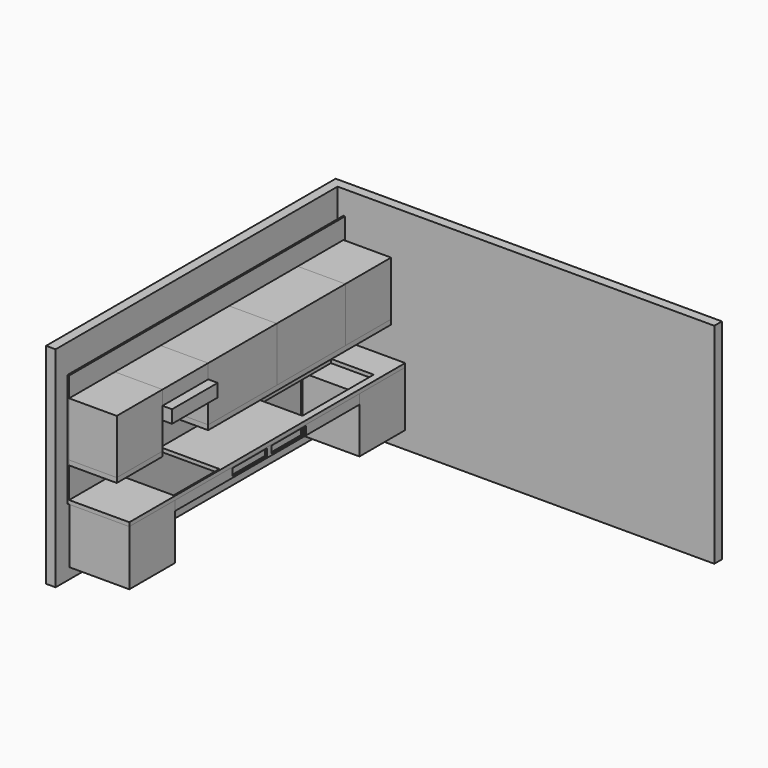
from build123d import *

# Parameters (mm, degrees)
F0_W      = 100
F0_H      = 3700
F1_DEPTH  = 2200
F2_W      = 650
F2_H      = 40
F3_DEPTH  = 3620
F4_W      = 18
F4_H      = 3620
F5_DEPTH  = 1150
F7_DEPTH  = 500
F6_W      = 900
F6_H      = 570
F8_DEPTH  = 500
F9_DEPTH  = 500
F6_W_2    = 600
F10_DEPTH = 500
F12_DEPTH = 630
F13_DEPTH = 600
F11_W     = 2420
F11_H     = 100
F14_DEPTH = 18
F15_W     = 18
F15_H     = 2420
F16_DEPTH = 600
F6_H_2    = 150
F17_DEPTH = 500
F6_H_3    = 135
F18_DEPTH = 600
F20_DEPTH = 50
F22_DEPTH = 50
F23_W     = 450
F23_H     = 75
F24_DEPTH = 25
F25_W     = 600
F25_H     = 600
F25_W_2   = 450
F25_H_2   = 450
F25_H_3   = 36.1033052649
F26_DEPTH = 50


with BuildPart() as f1:
    # F0 (on Top) → F1 (new body)
    with BuildSketch(Plane.XY):
        with Locations((-50, -1850)):
            Rectangle(F0_W, F0_H)
        Polygon((-100, 0), (0, 0), (3955.3870921059, 0), (3955.3870921059, 100), (-100, 100), align=None)
    extrude(amount=F1_DEPTH)


with BuildPart() as f3:
    # F2 (on face) → F3 (new body)
    with BuildSketch(Plane.XZ):
        with Locations((385, 780)):
            Rectangle(F2_W, F2_H)
    extrude(amount=F3_DEPTH)

    # F25 (on face) → F26 (cut)
    with BuildSketch(Plane.XY.offset(800)):
        with Locations((395, -2720)):
            Rectangle(F25_W, F25_H)
        with Locations((412.4879837036, -1032.7558462404)):
            Rectangle(F25_W_2, F25_H_2)
        with Locations((412.4879837036, -789.7041936079)):
            Rectangle(F25_W_2, F25_H_3)
        with Locations((412.4879837036, -546.6525409754)):
            Rectangle(F25_W_2, F25_H_2)
    extrude(amount=-F26_DEPTH, mode=Mode.SUBTRACT)


with BuildPart() as f5:
    # F4 (on face) → F5 (new body)
    with BuildSketch(Plane.XY.offset(800)):
        with Locations((69, -1810)):
            Rectangle(F4_W, F4_H)
    extrude(amount=F5_DEPTH)


with BuildPart() as f7:
    # F6 (on face) → F7 (new body)
    with BuildSketch(Plane.YZ.offset(78)):
        Polygon((-3020, 1740), (-3620, 1740), (-3620, 1170), (-3020, 1170), (-3020, 1455), (-3020, 1590), align=None)
    extrude(amount=F7_DEPTH)


with BuildPart() as f8:
    # F6 (on face) → F8 (new body)
    with BuildSketch(Plane.YZ.offset(78)):
        with Locations((-1070, 1455)):
            Rectangle(F6_W, F6_H)
    extrude(amount=F8_DEPTH)


with BuildPart() as f9:
    # F6 (on face) → F9 (new body)
    with BuildSketch(Plane.YZ.offset(78)):
        Polygon((-1520, 1740), (-2420, 1740), (-2420, 1590), (-2420, 1455), (-2420, 1170), (-1520, 1170), align=None)
    extrude(amount=F9_DEPTH)


with BuildPart() as f10:
    # F6 (on face) → F10 (new body)
    with BuildSketch(Plane.YZ.offset(78)):
        with Locations((-320, 1455)):
            Rectangle(F6_W_2, F6_H)
    extrude(amount=F10_DEPTH)


with BuildPart() as f12:
    # F11 (on face) → F12 (new body)
    with BuildSketch(Plane.YZ.offset(710)):
        Polygon((-3020, 760), (-3620, 760), (-3620, 180), (-3020, 180), (-3020, 660), align=None)
    extrude(amount=-F12_DEPTH)


with BuildPart() as f13:
    # F11 (on face) → F13 (new body)
    with BuildSketch(Plane.YZ.offset(710)):
        Polygon((0, 760), (-600, 760), (-600, 660), (-600, 180), (0, 180), align=None)
    extrude(amount=-F13_DEPTH)


with BuildPart() as f14:
    # F11 (on face) → F14 (new body)
    with BuildSketch(Plane.YZ.offset(710)):
        with Locations((-1810, 710)):
            Rectangle(F11_W, F11_H)
    extrude(amount=-F14_DEPTH)

    # F23 (on face) → F24 (cut)
    with BuildSketch(Plane.YZ.offset(710)):
        with Locations((-1529.4419670105, 712.5)):
            Rectangle(F23_W, F23_H)
        with Locations((-2039.4419670105, 712.5)):
            Rectangle(F23_W, F23_H)
    extrude(amount=-F24_DEPTH, mode=Mode.SUBTRACT)


with BuildPart() as f16:
    # F15 (on face) → F16 (new body)
    with BuildSketch(Plane(origin=(0, 0, 760), x_dir=(1, 0, 0), z_dir=(0, 0, -1))):
        with Locations((89, 1810)):
            Rectangle(F15_W, F15_H)
    extrude(amount=F16_DEPTH)


with BuildPart() as f17:
    # F6 (on face) → F17 (new body)
    with BuildSketch(Plane.YZ.offset(78)):
        with Locations((-2720, 1665)):
            Rectangle(F6_W_2, F6_H_2)
    extrude(amount=F17_DEPTH)


with BuildPart() as f18:
    # F6 (on face) → F18 (new body)
    with BuildSketch(Plane.YZ.offset(78)):
        with Locations((-2720, 1522.5)):
            Rectangle(F6_W_2, F6_H_3)
    extrude(amount=F18_DEPTH)


with BuildPart() as f20:
    # F19 (on face) → F20 (new body)
    with BuildSketch(Plane(origin=(0, 0, 1170), x_dir=(1, 0, 0), z_dir=(0, 0, -1))):
        Polygon((578, 3620), (78, 3620), (78, 3610), (568, 3610), (568, 3030), (78, 3030), (78, 3020), (578, 3020), align=None)
    extrude(amount=F20_DEPTH)


with BuildPart() as f22:
    # F21 (on face) → F22 (new body)
    with BuildSketch(Plane(origin=(0, 0, 1170), x_dir=(1, 0, 0), z_dir=(0, 0, -1))):
        Polygon((578, 2420), (78, 2420), (78, 2410), (568, 2410), (568, 30), (78, 30), (78, 20), (578, 20), align=None)
    extrude(amount=F22_DEPTH)


solid = Compound([f1.part, f3.part, f5.part, f7.part, f8.part, f9.part, f10.part, f12.part, f13.part, f14.part, f16.part, f17.part, f18.part, f20.part, f22.part])
